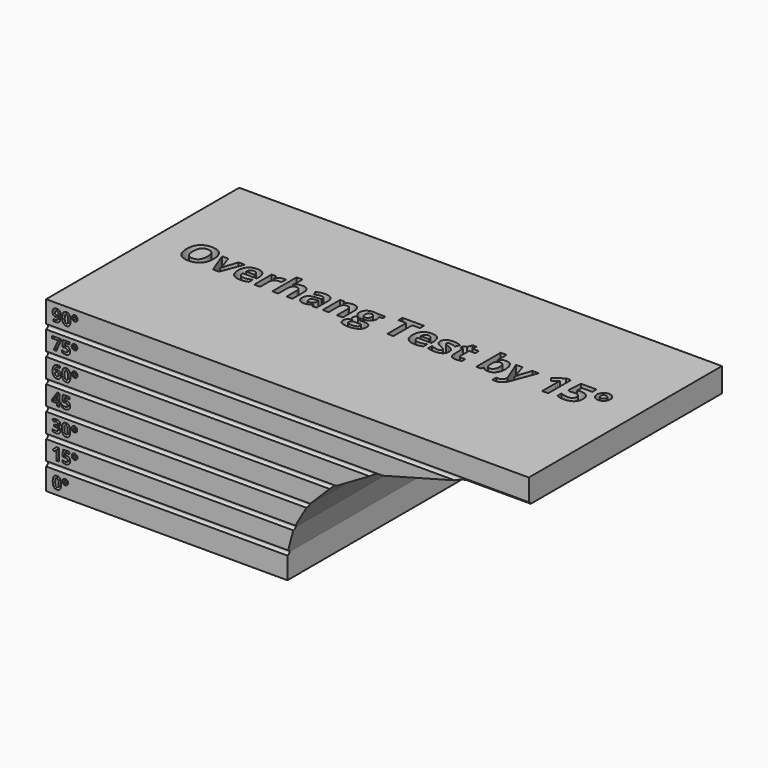
from build123d import *

# Parameters (mm, degrees)
F1_DEPTH     = 20
F3_DEPTH     = 40.001
F4_TEXT_SIZE = 1.3888888889
F5_DEPTH     = 0.5
F6_TEXT_SIZE = 3.3129723574
F7_DEPTH     = 1


# Not quite as in the source:
# - Text() gives the source's letters only with a copy of the font that has no kerning and outlines rounded to 1/6400 em; it was checked with that copy


with BuildPart() as f1:
    # F0 (on Front) → F1 (new body)
    with BuildSketch(Plane.XZ):
        Polygon((0, 14), (0, 0), (20, 0), (20, 2), (20.5358983849, 4), (21.6905989232, 6), (23.6905989232, 8), (27.1547005384, 10), (34.6188021535, 12), (40, 12), (40, 14), align=None)
    extrude(amount=F1_DEPTH)

    # F2 (on face) → F3 (cut, through all)
    with BuildSketch(Plane(origin=(0, 0, 0), x_dir=(0, -1, 0), z_dir=(-1, 0, 0))):
        with BuildLine():
            ThreePointArc((20, 10.2), (19.8, 10), (20, 9.8))
            Line((20, 9.8), (20, 10.2))
        make_face()
        with BuildLine():
            ThreePointArc((20, 8.2), (19.8, 8), (20, 7.8))
            Line((20, 7.8), (20, 8.2))
        make_face()
        with BuildLine():
            ThreePointArc((20, 6.2), (19.8, 6), (20, 5.8))
            Line((20, 5.8), (20, 6.2))
        make_face()
        with BuildLine():
            ThreePointArc((20, 4.2), (19.8, 4), (20, 3.8))
            Line((20, 3.8), (20, 4.2))
        make_face()
        with BuildLine():
            Line((20, 1.8), (20, 2.2))
            ThreePointArc((20, 2.2), (19.8, 2), (20, 1.8))
        make_face()
        with BuildLine():
            Line((20, 11.8), (20, 12.2))
            ThreePointArc((20, 12.2), (19.8, 12), (20, 11.8))
        make_face()
    extrude(amount=-F3_DEPTH, mode=Mode.SUBTRACT)

    # F4 (on face) → F5 (cut)
    with BuildSketch(Plane.XZ.offset(20)):
        with Locations((0.5, 0.4)):
            Text('0°', F4_TEXT_SIZE, font='Open Sans', font_style=FontStyle.BOLD, text_align=(TextAlign.LEFT, TextAlign.BOTTOM))
        with Locations((0.4800001043, 2.5)):
            Text('15°', F4_TEXT_SIZE, font='Open Sans', font_style=FontStyle.BOLD, text_align=(TextAlign.LEFT, TextAlign.BOTTOM))
        with Locations((0.4651561903, 4.5)):
            Text('30°', F4_TEXT_SIZE, font='Open Sans', font_style=FontStyle.BOLD, text_align=(TextAlign.LEFT, TextAlign.BOTTOM))
        with Locations((0.4660731647, 6.5)):
            Text('45', F4_TEXT_SIZE, font='Open Sans', font_style=FontStyle.BOLD, text_align=(TextAlign.LEFT, TextAlign.BOTTOM))
        with Locations((0.4846758675, 8.5)):
            Text('60°', F4_TEXT_SIZE, font='Open Sans', font_style=FontStyle.BOLD, text_align=(TextAlign.LEFT, TextAlign.BOTTOM))
        with Locations((0.4736430419, 10.5)):
            Text('75°', F4_TEXT_SIZE, font='Open Sans', font_style=FontStyle.BOLD, text_align=(TextAlign.LEFT, TextAlign.BOTTOM))
        with Locations((0.4946150584, 12.6)):
            Text('90°', F4_TEXT_SIZE, font='Open Sans', font_style=FontStyle.BOLD, text_align=(TextAlign.LEFT, TextAlign.BOTTOM))
    extrude(amount=-F5_DEPTH, mode=Mode.SUBTRACT)

    # F6 (on face) → F7 (cut)
    with BuildSketch(Plane.XY.offset(14)):
        with Locations((2.5, -10)):
            Text('Overhang Test by 15°', F6_TEXT_SIZE, font='Open Sans', font_style=FontStyle.BOLD, text_align=(TextAlign.LEFT, TextAlign.BOTTOM))
    extrude(amount=-F7_DEPTH, mode=Mode.SUBTRACT)


solid = f1.part
